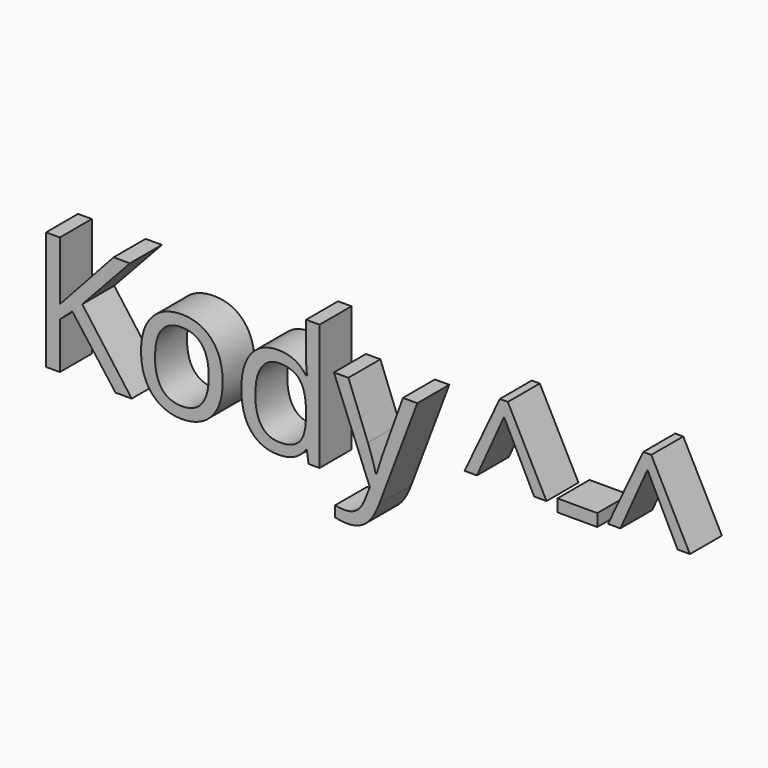
from build123d import *

# Parameters (mm, degrees)
F0_TEXT_SIZE = 211.0064754056
F1_DEPTH     = 50.8


# Not quite as in the source:
# - Text() gives the source's letters only with a copy of the font that has no kerning and outlines rounded to 1/6400 em; it was checked with that copy


with BuildPart() as f1:
    # F0 (on Front) → F1 (new body)
    with BuildSketch(Plane.XZ):
        with Locations((-76.2479007244, -75.9623274207)):
            Text('Kody ^-^', F0_TEXT_SIZE, font='Open Sans', text_align=(TextAlign.LEFT, TextAlign.BOTTOM))
    extrude(amount=F1_DEPTH)


solid = f1.part
